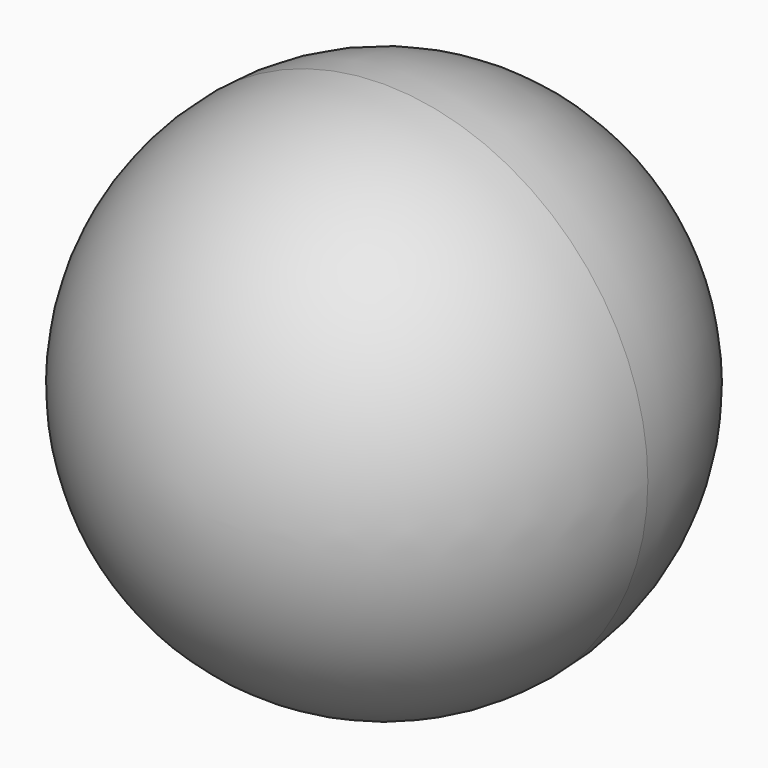
from build123d import *

# Parameters (mm, degrees)
F0_R     = 2.54
F1_DEPTH = 5.08
F2_R     = 2.54
F3_R     = 2.53999


# Not quite as in the source:
# - a fillet or chamfer is up to 0.001 mm smaller than in the source, because OpenCascade refuses the exact size


with BuildPart() as f1:
    # F0 (on Front) → F1 (new body)
    with BuildSketch(Plane.XZ):
        Circle(F0_R)
    extrude(amount=F1_DEPTH)

    # F2
    f2_edges = [f1.edges().sort_by_distance(p)[0] for p in [
        (-2.54, -5.08, 0),
    ]]
    fillet(f2_edges, radius=F2_R)

    # F3 (radius 2.54 in the source; OpenCascade refuses exactly that, so slightly less here)
    f3_edges = [f1.edges().sort_by_distance(p)[0] for p in [
        (-2.54, 0, 0),
    ]]
    fillet(f3_edges, radius=F3_R)


solid = f1.part
